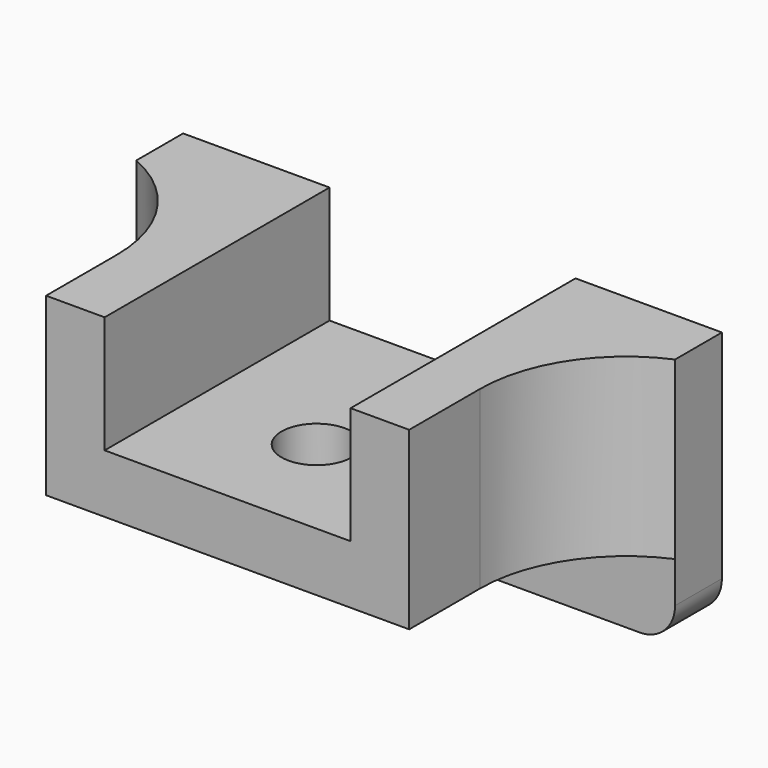
from build123d import *

# Parameters (mm, degrees)
F1_DEPTH    = 48
F2_DEPTH    = 10
F3_R        = 6
F4_T1_DEPTH = 30
F5_R        = 6
F6_DEPTH    = 3
F5_W        = 28
F5_H        = 5
F7_DEPTH    = 5
F8_DEPTH    = 25


# Not quite as in the source:
# - a fillet or chamfer that OpenCascade refuses, or shapes differently, is made with other operations: its cross-section is extruded or revolved along the edge and cut away or added


with BuildPart() as f1:
    # F0 (on Front) → F1 (new body)
    with BuildSketch(Plane.XZ):
        Polygon((-21, 43), (-31, 43), (-31, 13), (31, 13), (31, 43), (21, 43), (21, 23), (-21, 23), align=None)
    extrude(amount=F1_DEPTH)

    # F0 (on Front) → F2 (join)
    with BuildSketch(Plane.XZ):
        Polygon((-31, 43), (-46, 43), (-46, 0), (46, 0), (46, 43), (31, 43), (31, 13), (-31, 13), align=None)
        Polygon((-21, 43), (-31, 43), (-31, 13), (31, 13), (31, 43), (21, 43), (21, 23), (-21, 23), align=None)
    extrude(amount=F2_DEPTH)

    # F3
    f3_edges = [f1.edges().sort_by_distance(p)[0] for p in [
        (-46, -5, 0),
        (46, -5, 0),
    ]]
    fillet(f3_edges, radius=F3_R)

    # F4: fillet of radius 25 on 2 edges, made by hand

    # F4_s2 → F4_t1 (join)
    with BuildSketch(Plane.XY.offset(13)):
        with BuildLine():
            ThreePointArc((-46, -10), (-35.0834993366, -19.2198145372), (-31, -32.9128784748))
            Line((-31, -32.9128784748), (-31, -10))
            Line((-31, -10), (-46, -10))
        make_face()
        with BuildLine():
            ThreePointArc((46, -10), (35.0834993366, -19.2198145372), (31, -32.9128784748))
            Line((31, -32.9128784748), (31, -10))
            Line((31, -10), (46, -10))
        make_face()
    extrude(amount=F4_T1_DEPTH)

    # F5 (on face) → F6 (join)
    with BuildSketch(Plane(origin=(0, 0, 13), x_dir=(1, 0, 0), z_dir=(0, 0, -1))):
        with BuildLine():
            Line((14, 15), (14, 29))
            ThreePointArc((14, 29), (0, 43), (-14, 29))
            Line((-14, 29), (-14, 15))
            Line((-14, 15), (14, 15))
        make_face()
        with Locations((0, 29)):
            Circle(F5_R, mode=Mode.SUBTRACT)
    extrude(amount=F6_DEPTH)

    # F5 (on face) → F7 (join)
    with BuildSketch(Plane(origin=(0, 0, 13), x_dir=(1, 0, 0), z_dir=(0, 0, -1))):
        with Locations((0, 12.5)):
            Rectangle(F5_W, F5_H)
    extrude(amount=F7_DEPTH)

    # F5 (on face) → F8 (cut)
    with BuildSketch(Plane(origin=(0, 0, 13), x_dir=(1, 0, 0), z_dir=(0, 0, -1))):
        with Locations((0, 29)):
            Circle(F5_R)
    extrude(amount=-F8_DEPTH, mode=Mode.SUBTRACT)


solid = f1.part
